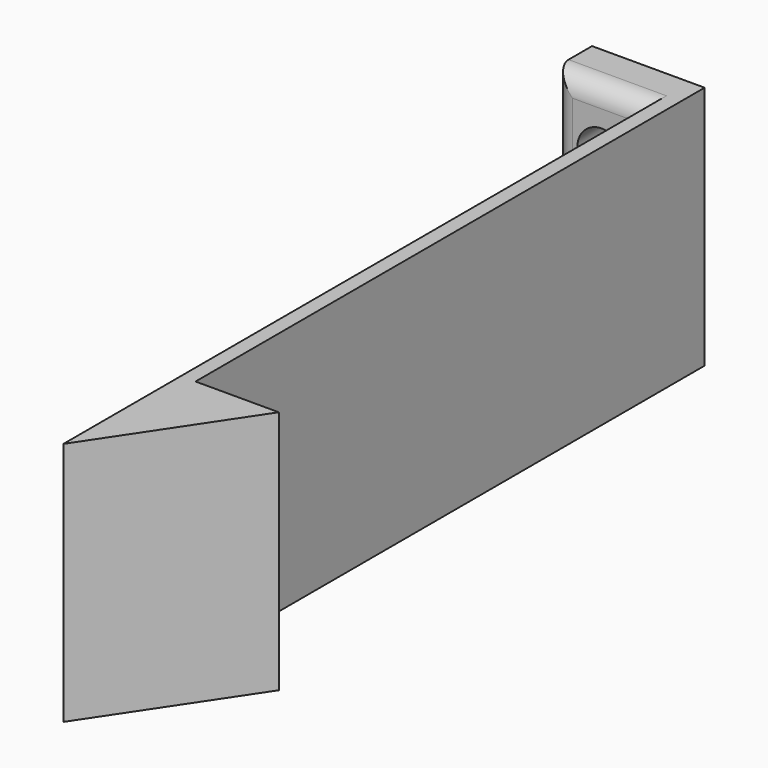
from build123d import *

# Parameters (mm, degrees)
F0_W     = 10
F0_H     = 5
F1_DEPTH = 25
F3_D     = 5
F4_R     = 2


# Not quite as in the source:
# - a feature names something its author has since deleted; it is built from what else it names


with BuildPart() as f1:
    # F0 (on Top) → F1 (new body)
    with BuildSketch(Plane.XY):
        Polygon((0, 60), (0, 0), (1.5, 0), (1.5, 65), (0, 65), align=None)
        with Locations((-5, 62.5)):
            Rectangle(F0_W, F0_H)
        Polygon((1.5, 0), (0, 0), (0, -15), (10, 0), align=None)
    extrude(amount=F1_DEPTH)

    # F3 (through all)
    with Locations(Plane.XZ.offset(-60)):
        with Locations((-5, 18.75), (-5, 6.25)):
            Hole(F3_D / 2)

    # F4
    f4_edges = [f1.edges().sort_by_distance(p)[0] for p in [
        (-10, 60, 12.5),
        (-5, 60, 25),
        (-5, 60, 0),
    ]]
    fillet(f4_edges, radius=F4_R)


solid = f1.part
